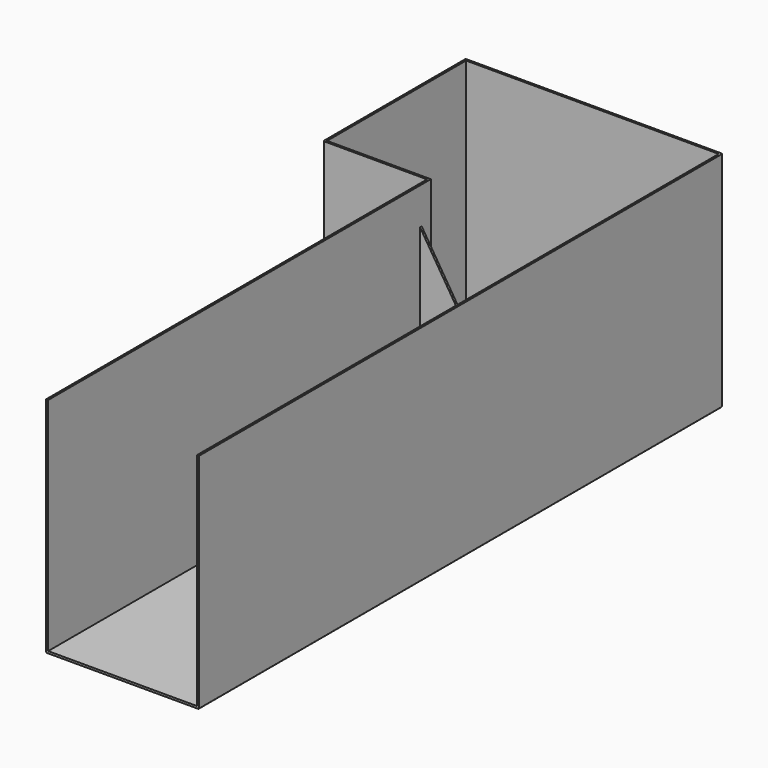
from build123d import *

# Parameters (mm, degrees)
F1_DEPTH  = 426
F3_DEPTH  = 4
F4_R      = 2
F7_DEPTH  = 4
F10_DEPTH = 4


# Not quite as in the source:
# - a feature names something its author has since deleted; it is built from what else it names


with BuildPart() as f1:
    # F0 (on Top) → F1 (new body)
    with BuildSketch(Plane.XY):
        Polygon((495, 0), (0, 0), (0, -343), (200, -343), (200, -1261), (204, -1261), (204, -339), (4, -339), (4, -4), (491, -4), (491, -1261), (495, -1261), align=None)
    extrude(amount=F1_DEPTH)

    # F2 (on Top) → F3 (join)
    with BuildSketch(Plane.XY):
        Polygon((0, -343), (200, -343), (199.9874711037, -1261), (495, -1261), (495, 0), (0, 0), align=None)
    extrude(amount=-F3_DEPTH)

    # F4
    f4_edges = [f1.edges().sort_by_distance(p)[0] for p in [
        (100, -343, -4),
        (0, -171.5, -4),
        (247.5, 0, -4),
        (0, -343, 211),
        (0, 0, 211),
        (495, 0, 211),
        (199.993736, -802, -4),
        (495, -630.5, -4),
    ]]
    fillet(f4_edges, radius=F4_R)

    # F6 (on offset) → F7 (join)
    with BuildSketch(Plane.XZ.offset(961)):
        Polygon((269, 0), (491, 0), (491, 355), align=None)
    extrude(amount=F7_DEPTH)

    # F9 (on offset) → F10 (join)
    with BuildSketch(Plane.XZ.offset(361)):
        Polygon((204, 355), (204, 0), (426, 0), align=None)
    extrude(amount=F10_DEPTH)


solid = f1.part
